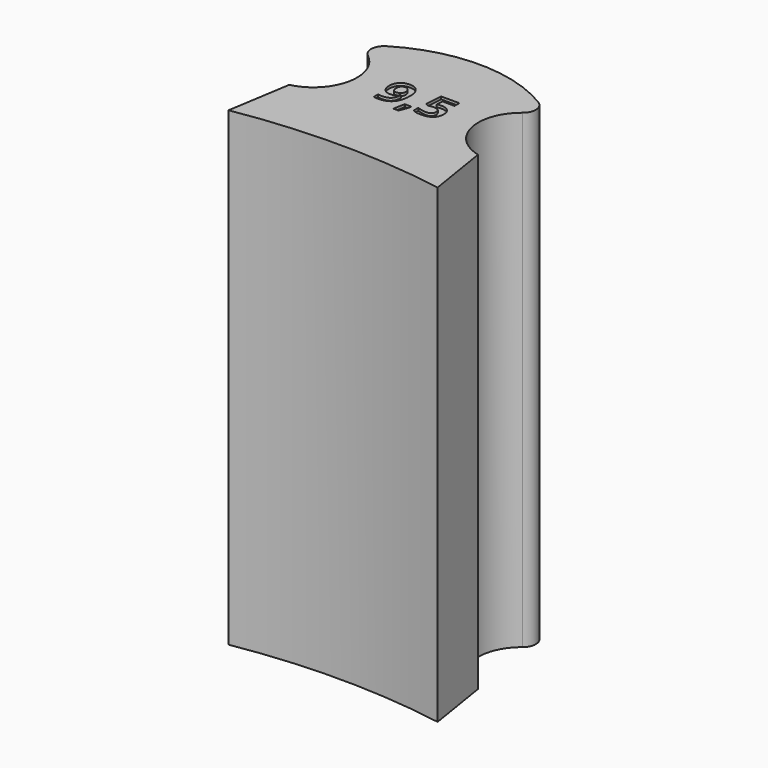
from build123d import *

# Parameters (mm, degrees)
F1_DEPTH     = 180
F2_TEXT_SIZE = 17.9236444334
F3_DEPTH     = 1


# Not quite as in the source:
# - Text() gives the source's letters only with a copy of the font that has no kerning and outlines rounded to 1/6400 em; it was checked with that copy


with BuildPart() as f1:
    # F0 (on Top) → F1 (new body)
    with BuildSketch(Plane.XY):
        with BuildLine():
            Line((3.8687128108, 24.1569802165), (0, 0))
            ThreePointArc((0, 0), (40, 3.356808676), (80, 0))
            Line((80, 0), (76.1312871892, 24.1569802165))
            ThreePointArc((76.1312871892, 24.1569802165), (63.5975554576, 36.8458138953), (69.5972800683, 53.6417728094))
            ThreePointArc((69.5972800683, 53.6417728094), (71.4969098635, 57.8715436357), (69.1043731597, 61.843359684))
            ThreePointArc((69.1043731597, 61.843359684), (40, 70), (10.8956268403, 61.843359684))
            ThreePointArc((10.8956268403, 61.843359684), (8.5030901365, 57.8715436357), (10.4027199317, 53.6417728094))
            ThreePointArc((10.4027199317, 53.6417728094), (16.4024445424, 36.8458138953), (3.8687128108, 24.1569802165))
        make_face()
    extrude(amount=F1_DEPTH)

    # F2 (on face) → F3 (cut)
    with BuildSketch(Plane.XY.offset(180)):
        with Locations((26.9913549386, 33.8757075369)):
            Text('9,5', F2_TEXT_SIZE, font='Open Sans', font_style=FontStyle.BOLD, text_align=(TextAlign.LEFT, TextAlign.BOTTOM))
    extrude(amount=-F3_DEPTH, mode=Mode.SUBTRACT)


solid = f1.part
